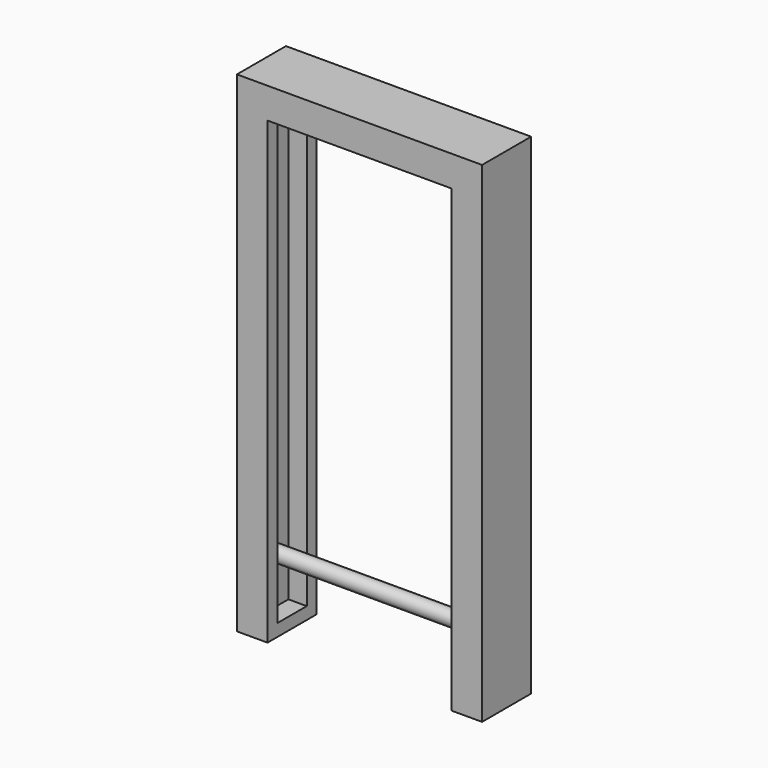
from build123d import *

# Parameters (mm, degrees)
F1_DEPTH = 12.7
F2_T     = -2.54
F3_R     = 1.5875418941
F4_DEPTH = 45.72


# Not quite as in the source:
# - a feature names something its author has since deleted; it is built from what else it names


with BuildPart() as f1:
    # F0 (on Front) → F1 (new body)
    with BuildSketch(Plane.XZ):
        Polygon((-105.322439312, 88.9), (-105.322439312, -12.7), (-98.972439312, -12.7), (-98.972439312, 0), (-98.972439312, 82.55), (-60.872439312, 82.55), (-60.872439312, 0), (-60.872439312, -12.7), (-54.522439312, -12.7), (-54.522439312, 88.9), align=None)
    extrude(amount=F1_DEPTH)

    # F2
    f2_openings = [f1.faces().sort_by_distance(p)[0] for p in [
        (-60.872439, -6.35, 34.925),
        (-79.922439, -6.35, 82.55),
        (-98.972439, -6.35, 34.925),
    ]]
    offset(amount=F2_T, openings=f2_openings)

    # F3 (on face) → F4 (join)
    with BuildSketch(Plane(origin=(-57.062439312, 0, 0), x_dir=(0, -1, 0), z_dir=(-1, 0, 0))):
        with Locations((6.2330360524, 0)):
            Circle(F3_R)
    extrude(amount=F4_DEPTH)


solid = f1.part
